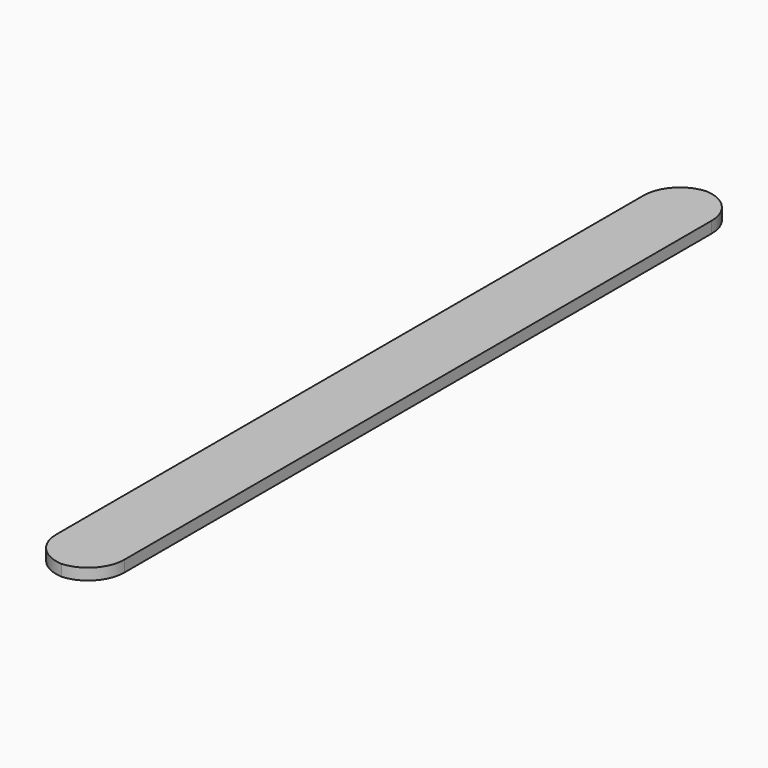
from build123d import *

# Parameters (mm, degrees)
F0_W        = 9.525
F0_H        = 112.7125
F1_DEPTH    = 1.5875
F2_T1_DEPTH = 26.9875


# Not quite as in the source:
# - a fillet or chamfer that OpenCascade refuses, or shapes differently, is made with other operations: its cross-section is extruded or revolved along the edge and cut away or added


with BuildPart() as f1:
    # F0 (on Top) → F1 (new body)
    with BuildSketch(Plane.XY):
        with Locations((0, 56.35625)):
            Rectangle(F0_W, F0_H)
    extrude(amount=F1_DEPTH)

    # F2: fillet of radius 5.08 on 4 edges, made by hand

    # F2_s2 → F2_t1 (cut)
    with BuildSketch(Plane.XY.offset(-12.7)):
        with BuildLine():
            ThreePointArc((-0.3175, 0), (3.2746024484, 1.4878975516), (4.7625, 5.08))
            Line((4.7625, 5.08), (4.7625, 0))
            Line((4.7625, 0), (-0.3175, 0))
        make_face()
        with BuildLine():
            ThreePointArc((-4.7625, 5.08), (-3.2746024484, 1.4878975516), (0.3175, 0))
            Line((0.3175, 0), (-4.7625, 0))
            Line((-4.7625, 0), (-4.7625, 5.08))
        make_face()
        with BuildLine():
            ThreePointArc((-0.3175, 112.7125), (3.2746024484, 111.2246024484), (4.7625, 107.6325))
            Line((4.7625, 107.6325), (4.7625, 112.7125))
            Line((4.7625, 112.7125), (-0.3175, 112.7125))
        make_face()
        with BuildLine():
            ThreePointArc((0.3175, 112.7125), (-3.2746024484, 111.2246024484), (-4.7625, 107.6325))
            Line((-4.7625, 107.6325), (-4.7625, 112.7125))
            Line((-4.7625, 112.7125), (0.3175, 112.7125))
        make_face()
    extrude(amount=F2_T1_DEPTH, mode=Mode.SUBTRACT)


solid = f1.part
